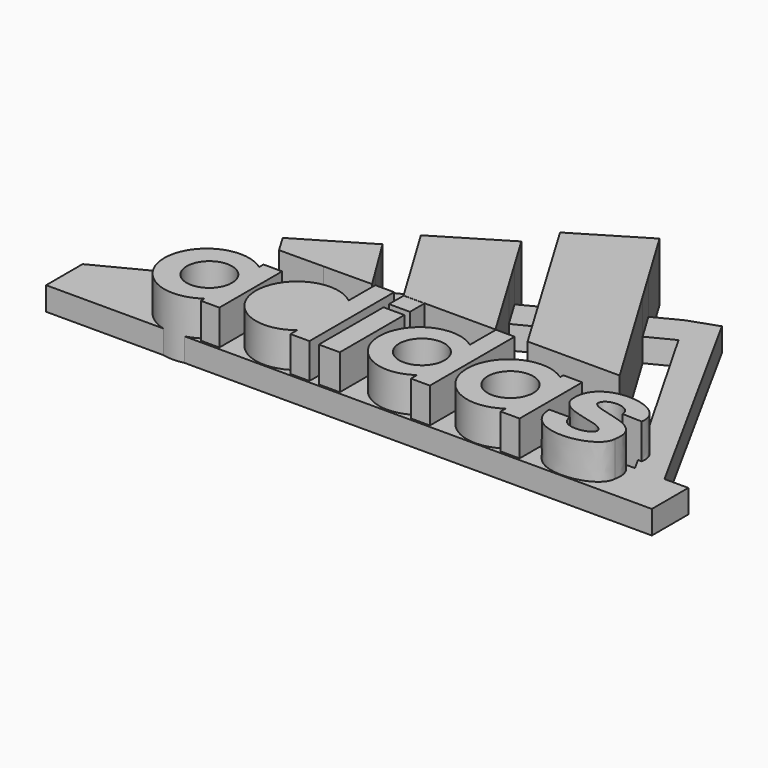
from build123d import *

# Parameters (mm, degrees)
F2_DEPTH = 25.4
F3_DEPTH = 10.16


# Not quite as in the source:
# - a feature names something its author has since deleted; it is built from what else it names


with BuildPart() as f2:
    # F1 (on Top) → F2 (new body)
    with BuildSketch(Plane.XY):
        with BuildLine():
            ThreePointArc((-63.7548551468, -58.759156792), (-63.6906221599, -58.1134173742), (-63.6691799498, -57.4648454785))
            ThreePointArc((-63.6691799498, -57.4648454785), (-63.6907839049, -56.8138346771), (-63.7555007085, -56.1656884515))
            Line((-63.7555007085, -56.1656884515), (-63.7548551468, -58.759156792))
        make_face()
        with BuildLine():
            ThreePointArc((-63.7555007085, -56.1656884515), (-63.6907839049, -56.8138346771), (-63.6691799498, -57.4648454785))
            ThreePointArc((-63.6691799498, -57.4648454785), (-63.6906221599, -58.1134173742), (-63.7548551468, -58.759156792))
            Line((-63.7548551468, -58.759156792), (-63.7514954563, -72.2563175644))
            ThreePointArc((-63.7514954563, -72.2563175644), (-58.247922708, -65.7524305272), (-56.2716146224, -57.4648454785))
            ThreePointArc((-56.2716146224, -57.4648454785), (-58.2499861473, -49.1731812372), (-63.7588605412, -42.6679562071))
            Line((-63.7588605412, -42.6679562071), (-63.7555007085, -56.1656884515))
        make_face()
        with BuildLine():
            ThreePointArc((-63.7548551468, -58.759156792), (-83.3082592689, -57.4672897417), (-63.7555007085, -56.1656884515))
            Line((-63.7555007085, -56.1656884515), (-63.7588605412, -42.6679562071))
            ThreePointArc((-63.7588605412, -42.6679562071), (-93.0016462367, -57.4694168672), (-63.7514954563, -72.2563175644))
            Line((-63.7514954563, -72.2563175644), (-63.7548551468, -58.759156792))
        make_face()
        with BuildLine():
            Line((-63.7594610453, -40.2555018663), (-63.7588605412, -42.6679562071))
            ThreePointArc((-63.7588605412, -42.6679562071), (-58.2499861473, -49.1731812372), (-56.2716146224, -57.4648454785))
            ThreePointArc((-56.2716146224, -57.4648454785), (-58.247922708, -65.7524305272), (-63.7514954563, -72.2563175644))
            Line((-63.7514954563, -72.2563175644), (-63.7509876773, -74.2962599682))
            Line((-63.7509876773, -74.2962599682), (-55.6843951345, -74.3069201708))
            Line((-55.6843951345, -74.3069201708), (-55.6843951345, -40.2555018663))
            Line((-55.6843951345, -40.2555018663), (-63.7594610453, -40.2555018663))
        make_face()
    extrude(amount=F2_DEPTH)



with BuildPart() as f2b:
    # F1 (on Top) → F2, piece 2 (new body)
    with BuildSketch(Plane.XY):
        with BuildLine():
            add(Edge.make_bspline(
                [(99.7076556087, -49.8992837965), (102.5500918428, -49.9901970228), (105.392528077, -50.081110249), (108.2349643111, -50.1720234752)],
                knots=[0, 0, 0, 0, 8.5316692763, 8.5316692763, 8.5316692763, 8.5316692763], degree=3))
            add(Edge.make_bspline(
                [(108.2349643111, -50.1720234752), (110.787704587, -36.6935394704), (79.6442404389, -33.426027745), (79.4406517156, -50.220690452)],
                knots=[0, 0, 0, 0, 28.7943537229, 28.7943537229, 28.7943537229, 28.7943537229], degree=3))
            add(Edge.make_bspline(
                [(79.4406517156, -50.220690452), (78.7407234311, -61.2938441336), (96.9160369831, -58.8432158298), (100.3960839706, -63.8056079812)],
                knots=[0, 0, 0, 0, 24.9735885541, 24.9735885541, 24.9735885541, 24.9735885541], degree=3))
            add(Edge.make_bspline(
                [(100.3960839706, -63.8056079812), (103.4537106752, -67.7798613906), (87.6547917724, -71.5578645468), (87.3998403549, -62.9053637385)],
                knots=[0, 0, 0, 0, 13.02738607, 13.02738607, 13.02738607, 13.02738607], degree=3))
            add(Edge.make_bspline(
                [(87.3998403549, -62.9053637385), (84.3765561779, -62.9053637385), (81.3532720009, -62.9053637385), (78.329987824, -62.9053637385)],
                knots=[0, 0, 0, 0, 9.069852531, 9.069852531, 9.069852531, 9.069852531], degree=3))
            add(Edge.make_bspline(
                [(78.329987824, -62.9053637385), (78.553237021, -80.3159624338), (108.8335961103, -76.5609592199), (109.1950891813, -65.7286011976)],
                knots=[0, 0, 0, 0, 30.9939534675, 30.9939534675, 30.9939534675, 30.9939534675], degree=3))
            add(Edge.make_bspline(
                [(109.1950891813, -65.7286011976), (111.9158491492, -51.4156892896), (91.7956531048, -54.4672831893), (88.140450418, -49.2563024163)],
                knots=[0, 0, 0, 0, 26.7326474669, 26.7326474669, 26.7326474669, 26.7326474669], degree=3))
            add(Edge.make_bspline(
                [(88.140450418, -49.2563024163), (88.1442502141, -43.7619574368), (99.8970344663, -44.0565347672), (99.7076556087, -49.8992837965)],
                knots=[0, 0, 0, 0, 11.5850619756, 11.5850619756, 11.5850619756, 11.5850619756], degree=3))
        make_face()
    extrude(amount=F2_DEPTH)


with BuildPart() as f2c:
    # F1 (on Top) → F2, piece 3 (new body)
    with BuildSketch(Plane.XY):
        with BuildLine():
            ThreePointArc((-24.7507108163, -58.9106234705), (-24.5838239541, -57.8642261235), (-24.527988285, -56.806076318))
            ThreePointArc((-24.527988285, -56.806076318), (-24.5827984166, -55.7576622945), (-24.7466312378, -54.7206787256))
            Line((-24.7466312378, -54.7206787256), (-24.7507108163, -58.9106234705))
        make_face()
        with BuildLine():
            ThreePointArc((-24.7466312378, -54.7206787256), (-24.5827984166, -55.7576622945), (-24.527988285, -56.806076318))
            ThreePointArc((-24.527988285, -56.806076318), (-24.5838239541, -57.8642261235), (-24.7507108163, -58.9106234705))
            Line((-24.7507108163, -58.9106234705), (-24.7622523782, -70.7644231243))
            ThreePointArc((-24.7622523782, -70.7644231243), (-19.8199434199, -64.5488407462), (-18.0565713242, -56.806076318))
            ThreePointArc((-18.0565713242, -56.806076318), (-19.8124122487, -49.0790081249), (-24.7350922441, -42.8695168514))
            Line((-24.7350922441, -42.8695168514), (-24.7466312378, -54.7206787256))
        make_face()
        with BuildLine():
            Line((-24.7507108163, -58.9106234705), (-24.7466312378, -54.7206787256))
            ThreePointArc((-24.7466312378, -54.7206787256), (-44.6369685256, -56.7962866728), (-24.7507108163, -58.9106234705))
        make_face()
        with BuildLine():
            ThreePointArc((-24.7507108163, -58.9106234705), (-44.6369685256, -56.7962866728), (-24.7466312378, -54.7206787256))
            Line((-24.7466312378, -54.7206787256), (-24.7350922441, -42.8695168514))
            ThreePointArc((-24.7350922441, -42.8695168514), (-53.8175246406, -56.7886668303), (-24.7622523782, -70.7644231243))
            Line((-24.7622523782, -70.7644231243), (-24.7507108163, -58.9106234705))
        make_face()
        with BuildLine():
            Line((-24.7210618109, -28.4595135599), (-24.7350922441, -42.8695168514))
            ThreePointArc((-24.7350922441, -42.8695168514), (-19.8124122487, -49.0790081249), (-18.0565713242, -56.806076318))
            ThreePointArc((-18.0565713242, -56.806076318), (-19.8199434199, -64.5488407462), (-24.7622523782, -70.7644231243))
            Line((-24.7622523782, -70.7644231243), (-24.7658085517, -74.4168029734))
            Line((-24.7658085517, -74.4168029734), (-16.501231119, -74.4141489267))
            Line((-16.501231119, -74.4141489267), (-16.501231119, -28.4595135599))
            Line((-16.501231119, -28.4595135599), (-24.7210618109, -28.4595135599))
        make_face()
    extrude(amount=F2_DEPTH)


with BuildPart() as f2d:
    # F1 (on Top) → F2, piece 4 (new body)
    with BuildSketch(Plane.XY):
        with BuildLine():
            ThreePointArc((27.5847475853, -53.826398746), (27.9304734188, -55.2984446386), (28.0466292686, -56.806076318))
            ThreePointArc((28.0466292686, -56.806076318), (27.9253867832, -58.3461648005), (27.5646464281, -59.8483094907))
            Line((27.5646464281, -59.8483094907), (27.5270910105, -71.0991728603))
            ThreePointArc((27.5270910105, -71.0991728603), (32.9193388863, -64.8381129636), (34.8593377287, -56.806076318))
            ThreePointArc((34.8593377287, -56.806076318), (32.946062473, -48.8263480127), (27.6222820027, -42.5818266111))
            Line((27.6222820027, -42.5818266111), (27.5847475853, -53.826398746))
        make_face()
        with BuildLine():
            ThreePointArc((27.5646464281, -59.8483094907), (8.3623938327, -56.7732233894), (27.5847475853, -53.826398746))
            Line((27.5847475853, -53.826398746), (27.6222820027, -42.5818266111))
            ThreePointArc((27.6222820027, -42.5818266111), (-0.335022445, -56.7473370387), (27.5270910105, -71.0991728603))
            Line((27.5270910105, -71.0991728603), (27.5646464281, -59.8483094907))
        make_face()
        with BuildLine():
            Line((27.6694223285, -28.4595135599), (27.6222820027, -42.5818266111))
            ThreePointArc((27.6222820027, -42.5818266111), (32.946062473, -48.8263480127), (34.8593377287, -56.806076318))
            ThreePointArc((34.8593377287, -56.806076318), (32.9193388863, -64.8381129636), (27.5270910105, -71.0991728603))
            Line((27.5270910105, -71.0991728603), (27.5160368181, -74.4107911787))
            Line((27.5160368181, -74.4107911787), (35.7560999691, -74.4168029734))
            Line((35.7560999691, -74.4168029734), (35.7560999691, -28.4595135599))
            Line((35.7560999691, -28.4595135599), (27.6694223285, -28.4595135599))
        make_face()
    extrude(amount=F2_DEPTH)


with BuildPart() as f2e:
    # F1 (on Top) → F2, piece 5 (new body)
    with BuildSketch(Plane.XY):
        with BuildLine():
            ThreePointArc((66.3250176765, -55.0119269433), (66.4481987929, -55.9052454716), (66.4893736218, -56.806076318))
            ThreePointArc((66.4893736218, -56.806076318), (66.4477565086, -57.7117222698), (66.3232559556, -58.609734623))
            Line((66.3232559556, -58.609734623), (66.3168991, -71.5917820143))
            ThreePointArc((66.3168991, -71.5917820143), (71.9428541009, -65.1303932452), (73.9693442177, -56.806076318))
            ThreePointArc((73.9693442177, -56.806076318), (71.9469282997, -48.4896360957), (66.3313741698, -42.0306194576))
            Line((66.3313741698, -42.0306194576), (66.3250176765, -55.0119269433))
        make_face()
        with BuildLine():
            ThreePointArc((66.3232559556, -58.609734623), (46.7396489921, -56.8012409428), (66.3250176765, -55.0119269433))
            Line((66.3250176765, -55.0119269433), (66.3313741698, -42.0306194576))
            ThreePointArc((66.3313741698, -42.0306194576), (37.7486345832, -56.7972083097), (66.3168991, -71.5917820143))
            Line((66.3168991, -71.5917820143), (66.3232559556, -58.609734623))
        make_face()
        with BuildLine():
            Line((66.3322433829, -40.2555018663), (66.3313741698, -42.0306194576))
            ThreePointArc((66.3313741698, -42.0306194576), (71.9469282997, -48.4896360957), (73.9693442177, -56.806076318))
            ThreePointArc((73.9693442177, -56.806076318), (71.9428541009, -65.1303932452), (66.3168991, -71.5917820143))
            Line((66.3168991, -71.5917820143), (66.3155749377, -74.2960021653))
            Line((66.3155749377, -74.2960021653), (74.5772473478, -74.3069201708))
            Line((74.5772473478, -74.3069201708), (74.5772473478, -40.3231311066))
            Line((74.5772473478, -40.3231311066), (66.3322433829, -40.2555018663))
        make_face()
    extrude(amount=F2_DEPTH)


with BuildPart() as f2f:
    # F1 (on Top) → F2, piece 6 (new body)
    with BuildSketch(Plane.XY):
        Polygon((-3.3386279955, -39.3958377083), (-12.4006029218, -39.3581949174), (-12.4518834054, -74.4168029734), (-3.3386279955, -74.4168029734), align=None)
    extrude(amount=F2_DEPTH)


with BuildPart() as f2g:
    # F1 (on Top) → F2, piece 7 (new body)
    with BuildSketch(Plane.XY):
        Polygon((-3.3386279955, -28.4714891851), (-12.4006029218, -28.4595135599), (-12.4006029218, -36.3864824176), (-3.3386279955, -36.3864824176), align=None)
    extrude(amount=F2_DEPTH)


with BuildPart() as f2h:
    # F0 (on Top) → F2, piece 8 (new body)
    with BuildSketch(Plane.XY):
        Polygon((-41.548015992, -3.4748504169), (-70.8924457431, -20.9543742239), (-69.0594983918, -24.0315058084), (-38.5506476001, -8.3180443033), align=None)
        Polygon((-38.5506476001, -8.3180443033), (-69.0594983918, -24.0315058084), (-66.2418976426, -28.7616625428), (-47.085140646, -28.6405240715), (-31.034172326, -20.4632805027), align=None)
        Polygon((-31.034172326, -20.4632805027), (-47.085140646, -28.6405240715), (-26.0557178408, -28.5075437278), align=None)
    extrude(amount=F2_DEPTH)


with BuildPart() as f2i:
    # F0 (on Top) → F2, piece 9 (new body)
    with BuildSketch(Plane.XY):
        Polygon((2.6448233617, 12.899518153), (-27.9053643064, -2.8352337449), (-20.5059778619, -15.0996408296), (10.0803808061, 0.4827277681), align=None)
        Polygon((-35.5255827308, 9.7952000797), (-27.9053643064, -2.8352337449), (2.6448233617, 12.899518153), (-6.1135631986, 27.5253280997), align=None)
        Polygon((10.0803808061, 0.4827277681), (-20.5059778619, -15.0996408296), (-12.4883763492, -28.3887330443), (27.3695029318, -28.3887330443), align=None)
    extrude(amount=F2_DEPTH)


with BuildPart() as f2j:
    # F0 (on Top) → F2, piece 10 (new body)
    with BuildSketch(Plane.XY):
        Polygon((43.7538640592, 34.0725650476), (13.3862376873, 18.4318406148), (20.8315235803, 5.9599495378), (51.3153258259, 21.4900702692), align=None)
        Polygon((0, 40.855653584), (13.3862376873, 18.4318406148), (43.7538640592, 34.0725650476), (29.1310697794, 58.4053248167), align=None)
        Polygon((81.3401341438, -28.4720938653), (51.3153258259, 21.4900702692), (20.8315235803, 5.9599495378), (41.3862578571, -28.4720938653), align=None)
    extrude(amount=F2_DEPTH)


with BuildPart() as f2_1:
    add(f2.part)

    add(f2b.part)  # F3 merges F2b

    add(f2c.part)  # F3 merges F2c

    add(f2d.part)  # F3 merges F2d

    add(f2e.part)  # F3 merges F2e

    add(f2f.part)  # F3 merges F2f

    add(f2h.part)  # F3 merges F2h

    add(f2i.part)  # F3 merges F2i

    add(f2j.part)  # F3 merges F2j
    # F0 (on Top) → F3 (join)
    with BuildSketch(Plane.XY):
        Polygon((62.3871354147, 27.1306573011), (109.6180081367, -55.4669238627), (122.3754435778, -55.4669238627), (67.5358325243, 44.2334525287), (54.7744184732, 39.7486574948), align=None)
        Polygon((51.3153258259, 21.4900702692), (62.3871354147, 27.1306573011), (54.7744184732, 39.7486574948), (43.7538640592, 34.0725650476), align=None)
        Polygon((-66.2418976426, -28.7616625428), (-69.0594983918, -24.0315058084), (-130.0936937332, -55.4669238627), (-99.7422114015, -55.4669238627), (-47.085140646, -28.6405240715), align=None)
        Polygon((-27.9053643064, -2.8352337449), (-38.5506476001, -8.3180443033), (-31.034172326, -20.4632805027), (-20.5059778619, -15.0996408296), align=None)
        Polygon((13.3862376873, 18.4318406148), (2.6448233617, 12.899518153), (10.0803808061, 0.4827277681), (20.8315235803, 5.9599495378), align=None)
        Polygon((-99.7422114015, -55.4669238627), (-130.0936937332, -55.4669238627), (-130.0936937332, -75.2655499159), (-91.6557535529, -75.2655499159), (132.7225416899, -75.2655499159), (132.7225416899, -55.4669238627), (122.3754435778, -55.4669238627), (109.6180081367, -55.4669238627), align=None)
    extrude(amount=F3_DEPTH)


solid = Compound([f2g.part, f2_1.part])
